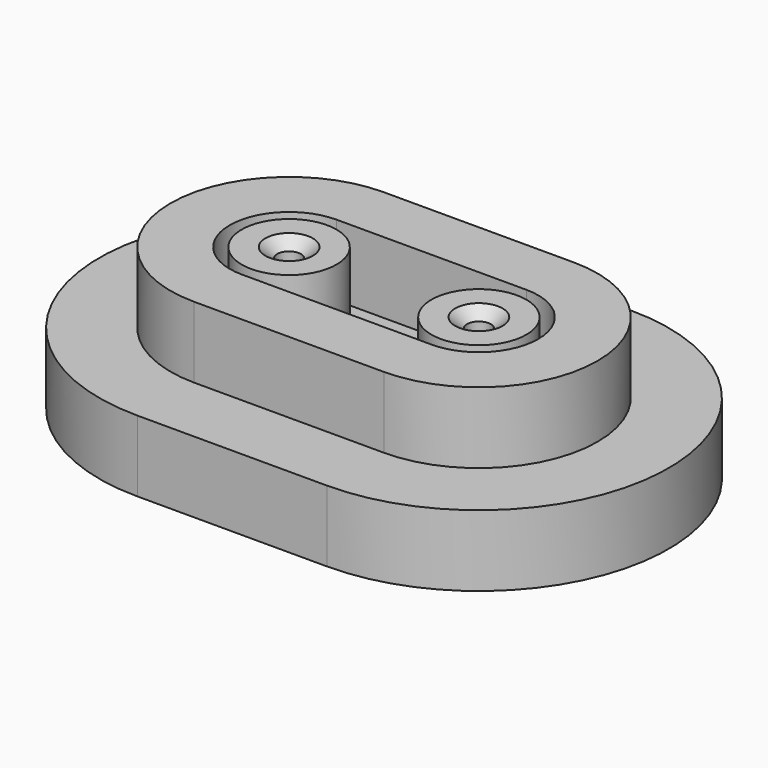
from build123d import *

# Parameters (mm, degrees)
F0_R           = 50.8
F0_R_2         = 25.4
F1_DEPTH       = 76.2
F2_DEPTH       = 152.4
F4_DEPTH       = 25.4
F6_D           = 25.4
F6_CSINK_D     = 50.8
F6_CSINK_ANGLE = 100


# Not quite as in the source:
# - a feature names something its author has since deleted; it is built from what else it names


with BuildPart() as f1:
    # F0 (on Top) → F1 (new body)
    with BuildSketch(Plane.XY):
        with BuildLine():
            Line((101.6, 203.2), (-101.6, 203.2))
            ThreePointArc((-101.6, 203.2), (-304.8, 0), (-101.6, -203.2))
            Line((-101.6, -203.2), (101.6, -203.2))
            ThreePointArc((101.6, -203.2), (304.8, 0), (101.6, 203.2))
        make_face()
        with BuildLine():
            ThreePointArc((-101.6, -127), (-228.6, 0), (-101.6, 127))
            Line((-101.6, 127), (101.6, 127))
            ThreePointArc((101.6, 127), (228.6, 0), (101.6, -127))
            Line((101.6, -127), (-101.6, -127))
        make_face(mode=Mode.SUBTRACT)
        with BuildLine():
            Line((101.6, 127), (-101.6, 127))
            ThreePointArc((-101.6, 127), (-228.6, 0), (-101.6, -127))
            Line((-101.6, -127), (101.6, -127))
            ThreePointArc((101.6, -127), (228.6, 0), (101.6, 127))
        make_face()
        with BuildLine():
            ThreePointArc((101.6, 63.5), (165.1, 0), (101.6, -63.5))
            Line((101.6, -63.5), (-101.6, -63.5))
            ThreePointArc((-101.6, -63.5), (-165.1, 0), (-101.6, 63.5))
            Line((-101.6, 63.5), (101.6, 63.5))
        make_face(mode=Mode.SUBTRACT)
        with BuildLine():
            Line((-101.6, -63.5), (101.6, -63.5))
            ThreePointArc((101.6, -63.5), (165.1, 0), (101.6, 63.5))
            Line((101.6, 63.5), (-101.6, 63.5))
            ThreePointArc((-101.6, 63.5), (-165.1, 0), (-101.6, -63.5))
        make_face()
        with Locations((-101.6, 0)):
            Circle(F0_R, mode=Mode.SUBTRACT)
        with Locations((101.6, 0)):
            Circle(F0_R, mode=Mode.SUBTRACT)
        with Locations((-101.6, 0)):
            Circle(F0_R)
        with Locations((-101.6, 0)):
            Circle(F0_R_2, mode=Mode.SUBTRACT)
        with Locations((101.6, 0)):
            Circle(F0_R)
        with Locations((101.6, 0)):
            Circle(F0_R_2, mode=Mode.SUBTRACT)
        with Locations((-101.6, 0)):
            Circle(F0_R_2)
        with Locations((101.6, 0)):
            Circle(F0_R_2)
    extrude(amount=F1_DEPTH)

    # F0 (on Top) → F2 (join)
    with BuildSketch(Plane.XY):
        with BuildLine():
            Line((101.6, 127), (-101.6, 127))
            ThreePointArc((-101.6, 127), (-228.6, 0), (-101.6, -127))
            Line((-101.6, -127), (101.6, -127))
            ThreePointArc((101.6, -127), (228.6, 0), (101.6, 127))
        make_face()
        with BuildLine():
            ThreePointArc((101.6, 63.5), (165.1, 0), (101.6, -63.5))
            Line((101.6, -63.5), (-101.6, -63.5))
            ThreePointArc((-101.6, -63.5), (-165.1, 0), (-101.6, 63.5))
            Line((-101.6, 63.5), (101.6, 63.5))
        make_face(mode=Mode.SUBTRACT)
        with Locations((101.6, 0)):
            Circle(F0_R)
        with Locations((101.6, 0)):
            Circle(F0_R_2, mode=Mode.SUBTRACT)
        with Locations((-101.6, 0)):
            Circle(F0_R)
        with Locations((-101.6, 0)):
            Circle(F0_R_2, mode=Mode.SUBTRACT)
        with Locations((101.6, 0)):
            Circle(F0_R_2)
        with Locations((-101.6, 0)):
            Circle(F0_R_2)
    extrude(amount=F2_DEPTH)

    # F3 (on face) → F4 (cut)
    with BuildSketch(Plane.XY):
        with BuildLine():
            Line((101.6, 101.6), (-101.6, 101.6))
            ThreePointArc((-101.6, 101.6), (-203.2, 0), (-101.6, -101.6))
            Line((-101.6, -101.6), (101.6, -101.6))
            ThreePointArc((101.6, -101.6), (203.2, 0), (101.6, 101.6))
        make_face()
    extrude(amount=F4_DEPTH, mode=Mode.SUBTRACT)

    # F6 (through all)
    with Locations(Plane.XY.offset(152.4)):
        with Locations((-101.6, 0), (101.6, 0)):
            CounterSinkHole(F6_D / 2, F6_CSINK_D / 2, counter_sink_angle=F6_CSINK_ANGLE)


solid = f1.part
